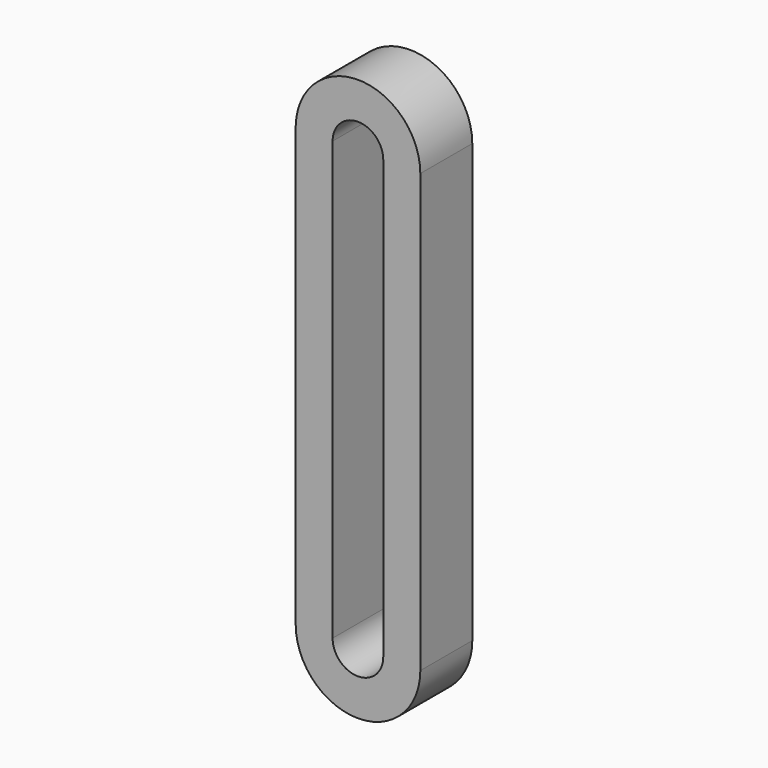
from build123d import *

# Parameters (mm, degrees)
F1_DEPTH = 2.286
F2_D     = 1.778


with BuildPart() as f1:
    # F0 (on Front) → F1 (new body)
    with BuildSketch(Plane.XZ):
        with BuildLine():
            ThreePointArc((-44.9743270874, 48.1504499912), (-47.139991973, 50.3428364156), (-49.3587702513, 48.2042187354))
            Line((-49.3587702513, 48.2042187354), (-49.3587702513, 32.7516756952))
            ThreePointArc((-49.3587702513, 32.7516756952), (-47.1665486693, 30.5594541132), (-44.9743270874, 32.7516756952))
            Line((-44.9743270874, 32.7516756952), (-44.9743270874, 48.1504499912))
        make_face()
        with BuildLine():
            ThreePointArc((-48.060906813, 48.1504499912), (-47.1693925898, 49.0419642144), (-46.2778783666, 48.1504499912))
            Line((-46.2778783666, 48.1504499912), (-46.2778783666, 32.7516756952))
            ThreePointArc((-46.2778783666, 32.7516756952), (-47.1693925898, 31.860161472), (-48.060906813, 32.7516756952))
            Line((-48.060906813, 32.7516756952), (-48.060906813, 48.1504499912))
        make_face(mode=Mode.SUBTRACT)
    extrude(amount=F1_DEPTH)

    # F2 (through all)
    with Locations(Plane(origin=(0, 0, 0), x_dir=(1, 0, 0), z_dir=(0, 1, 0))):
        with Locations((-47.1668783666, -48.1504499912), (-47.1665486693, -32.7516756952)):
            Hole(F2_D / 2)


solid = f1.part
